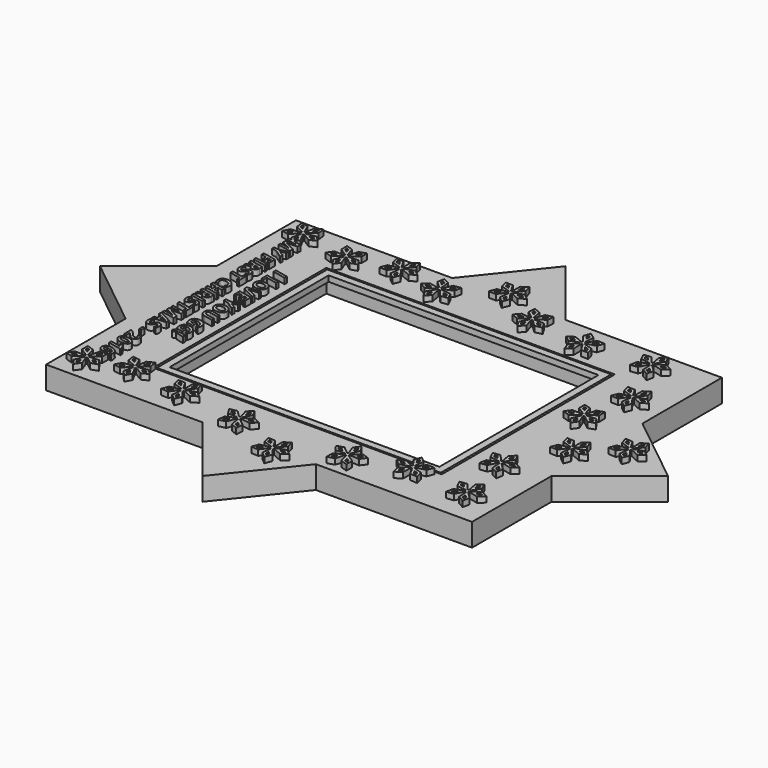
from build123d import *

# Parameters (mm, degrees)
F1_DEPTH     = 4
F4_W         = 101.6
F4_H         = 76.2
F5_DEPTH     = 8.001
F6_DEPTH     = 2
F7_TEXT_SIZE = 6.5647362641
F8_DEPTH     = 2
F9_W         = 100
F9_H         = 75
F9_W_2       = 95
F9_H_2       = 70
F10_DEPTH    = 2


# Not quite as in the source:
# - Text() gives the source's letters only with a copy of the font that has no kerning and outlines rounded to 1/6400 em; it was checked with that copy


with BuildPart() as f1:
    # F0 (on Top) → F1 (new body, symmetric)
    with BuildSketch(Plane.XY):
        Polygon((75, 20), (75, 55), (20, 55), (0, 80), (-20, 55), (-75, 55), (-75, 20), (-100, 0), (-75, -20), (-75, -55), (-20, -55), (0, -80), (20, -55), (75, -55), (75, -20), (100, 0), align=None)
    extrude(amount=F1_DEPTH, both=True)

    # F4 (on face) → F5 (cut, through all)
    with BuildSketch(Plane.XY.offset(4)):
        Rectangle(F4_W, F4_H)
    extrude(amount=-F5_DEPTH, mode=Mode.SUBTRACT)

    # F2 (on face) → F6 (join)
    with BuildSketch(Plane.XY.offset(4)):
        with BuildLine():
            Line((63.1994701679, 31.4178951368), (60.6442793174, 31.5524958216))
            Line((60.6442793174, 31.5524958216), (61.3153708432, 29.0833352779))
            Line((61.3153708432, 29.0833352779), (64.6001066479, 28.016059918))
            ThreePointArc((64.6001066479, 28.016059918), (64.5643629359, 27.8223093015), (64.5803085929, 27.6259355498))
            Line((64.5803085929, 27.6259355498), (61.2044020685, 26.8966748697))
            Line((61.2044020685, 26.8966748697), (60.2867918134, 24.5081378601))
            Line((60.2867918134, 24.5081378601), (62.8424817245, 24.3833712589))
            Line((62.8424817245, 24.3833712589), (64.8725600959, 27.1775344264))
            ThreePointArc((64.8725600959, 27.1775344264), (65.0457824678, 27.083667903), (65.237472483, 27.0381502975))
            Line((65.237472483, 27.0381502975), (64.8878281174, 23.6021184556))
            Line((64.8878281174, 23.6021184556), (66.8759046418, 21.9913207154))
            Line((66.8759046418, 21.9913207154), (67.7843163458, 24.3833712589))
            Line((67.7843163458, 24.3833712589), (65.7542379744, 27.1775344264))
            ThreePointArc((65.7542379744, 27.1775344264), (65.8970389999, 27.313272341), (65.9995642876, 27.4815146655))
            Line((65.9995642876, 27.4815146655), (69.15937871, 26.0871908808))
            Line((69.15937871, 26.0871908808), (71.3056878294, 27.480200138))
            Line((71.3056878294, 27.480200138), (69.3114272272, 29.0833352779))
            Line((69.3114272272, 29.0833352779), (66.0266914224, 28.016059918))
            ThreePointArc((66.0266914224, 28.016059918), (65.9417249379, 28.1938170862), (65.8133990352, 28.3433141666))
            Line((65.8133990352, 28.3433141666), (68.115916112, 30.9176065182))
            Line((68.115916112, 30.9176065182), (67.4543315738, 33.389331326))
            Line((67.4543315738, 33.389331326), (65.3133990352, 31.9880727875))
            Line((65.3133990352, 31.9880727875), (65.3133990352, 28.5342971722))
            ThreePointArc((65.3133990352, 28.5342971722), (65.1180858343, 28.5084192293), (64.9362507771, 28.4325711818))
            Line((64.9362507771, 28.4325711818), (63.1994701679, 31.4178951368))
        make_face()
        Polygon((62.2964551725, 25.2211391292), (61.4445585355, 25.2627279962), (61.7504286205, 26.0589069994), (63.1200942761, 26.3547811003), align=None, mode=Mode.SUBTRACT)
        Polygon((66.8188202697, 24.1229536578), (66.5160163683, 23.3256034766), (65.8533241935, 23.8625360567), (65.9951811661, 25.2565956289), align=None, mode=Mode.SUBTRACT)
        Polygon((69.2607769989, 28.0852630793), (69.9263859742, 27.5501970319), (69.2100289384, 27.0852630793), (67.9263859742, 27.6516931529), align=None, mode=Mode.SUBTRACT)
        Polygon((61.9434039514, 29.8615218975), (61.7197067761, 30.6845754121), (62.5714370596, 30.6397085171), (63.2760800154, 29.4285091956), align=None, mode=Mode.SUBTRACT)
        Polygon((66.2475713941, 31.6312506978), (66.9612155737, 32.0983368772), (67.1817437531, 31.274428608), (66.2475713941, 30.2299921593), align=None, mode=Mode.SUBTRACT)
        with BuildLine():
            Line((60.4743340463, 15.1066376163), (58.0410464334, 15.89798395))
            Line((58.0410464334, 15.89798395), (58.0502052958, 13.3392667437))
            Line((58.0502052958, 13.3392667437), (60.9467852527, 11.4582057254))
            ThreePointArc((60.9467852527, 11.4582057254), (60.8621131286, 11.2803081545), (60.8266901836, 11.0864986364))
            Line((60.8266901836, 11.0864986364), (57.3770683317, 11.2558358144))
            Line((57.3770683317, 11.2558358144), (55.8725260198, 9.1861812398))
            Line((55.8725260198, 9.1861812398), (58.3088409363, 8.404204735))
            Line((58.3088409363, 8.404204735), (60.9929287076, 10.5777361558))
            ThreePointArc((60.9929287076, 10.5777361558), (61.1359542263, 10.4422348077), (61.3093317395, 10.3486551503))
            Line((61.3093317395, 10.3486551503), (60.0822907364, 7.1201978751))
            Line((60.0822907364, 7.1201978751), (61.585720063, 5.0497346693))
            Line((61.585720063, 5.0497346693), (63.0822866263, 7.1251638173))
            Line((63.0822866263, 7.1251638173), (61.8445641408, 10.3495411293))
            ThreePointArc((61.8445641408, 10.3495411293), (62.0176308968, 10.4436942615), (62.1602070378, 10.5796683707))
            Line((62.1602070378, 10.5796683707), (64.8514758442, 8.4150348653))
            Line((64.8514758442, 8.4150348653), (67.2851885796, 9.2050728063))
            Line((67.2851885796, 9.2050728063), (65.7738026656, 11.2697350658))
            Line((65.7738026656, 11.2697350658), (62.3247603297, 11.0889784163))
            ThreePointArc((62.3247603297, 11.0889784163), (62.2886959485, 11.2826696003), (62.2034353365, 11.4602858788))
            Line((62.2034353365, 11.4602858788), (65.0937719348, 13.3509260745))
            Line((65.0937719348, 13.3509260745), (65.0944597975, 15.9096595802))
            Line((65.0944597975, 15.9096595802), (62.6638053693, 15.1102618839))
            Line((62.6638053693, 15.1102618839), (61.7699024625, 11.7741708188))
            ThreePointArc((61.7699024625, 11.7741708188), (61.5745466931, 11.7997254216), (61.379276596, 11.7735242095))
            Line((61.379276596, 11.7735242095), (60.4743340463, 15.1066376163))
        make_face()
        Polygon((57.9982500681, 9.3547484281), (57.1861450959, 9.6154072631), (57.6876591999, 10.3052921213), (59.0872324822, 10.2365889995), align=None, mode=Mode.SUBTRACT)
        Polygon((58.8582482127, 13.9283903679), (58.8551952585, 14.7812961033), (59.6662911295, 14.5175139921), (60.0334425069, 13.1652102697), align=None, mode=Mode.SUBTRACT)
        Polygon((62.0822879963, 7.1235085032), (61.5834324752, 6.4316987872), (61.0822893664, 7.1218531892), (61.5801218471, 8.4316960472), align=None, mode=Mode.SUBTRACT)
        Polygon((65.4665582086, 10.3187805964), (65.9710018247, 9.6296742031), (65.1587203012, 9.3659893347), (64.0654193012, 10.2453500178), align=None, mode=Mode.SUBTRACT)
        Polygon((63.4737942244, 14.5238166141), (64.2840123672, 14.7902825129), (64.2837830796, 13.9373713443), (63.1111218276, 13.1703048025), align=None, mode=Mode.SUBTRACT)
        with BuildLine():
            Line((54.531646123, 49.5059511711), (51.9919011994, 49.1948027344))
            Line((51.9919011994, 49.1948027344), (53.0815625657, 46.879688108))
            Line((53.0815625657, 46.879688108), (56.5017262742, 46.3990154456))
            ThreePointArc((56.5017262742, 46.3990154456), (56.5001700309, 46.2020015058), (56.5499733817, 46.0113800469))
            Line((56.5499733817, 46.0113800469), (53.3519892511, 44.7069784593))
            Line((53.3519892511, 44.7069784593), (52.8630846567, 42.1953873453))
            Line((52.8630846567, 42.1953873453), (55.4016133884, 42.5163071248))
            Line((55.4016133884, 42.5163071248), (56.9156489656, 45.6205400851))
            ThreePointArc((56.9156489656, 45.6205400851), (57.1025394512, 45.5581793543), (57.2992213136, 45.5466398853))
            Line((57.2992213136, 45.5466398853), (57.5515494993, 42.1020939809))
            Line((57.5515494993, 42.1020939809), (59.7891347663, 40.8609937433))
            Line((59.7891347663, 40.8609937433), (60.2683704375, 43.3744477011))
            Line((60.2683704375, 43.3744477011), (57.783932176, 45.773641842))
            ThreePointArc((57.783932176, 45.773641842), (57.9009930915, 45.9321147305), (57.9727458167, 46.1156044054))
            Line((57.9727458167, 46.1156044054), (61.3266773423, 45.2911595482))
            Line((61.3266773423, 45.2911595482), (63.1984856844, 47.035708532))
            Line((63.1984856844, 47.035708532), (60.9561408862, 48.2681887276))
            Line((60.9561408862, 48.2681887276), (57.9066380204, 46.6467392919))
            ThreePointArc((57.9066380204, 46.6467392919), (57.7920951594, 46.8070416542), (57.6397589199, 46.9319839788))
            Line((57.6397589199, 46.9319839788), (59.460274413, 49.8669949397))
            Line((59.460274413, 49.8669949397), (58.3795303219, 52.1862857442))
            Line((58.3795303219, 52.1862857442), (56.5144493508, 50.4345464378))
            Line((56.5144493508, 50.4345464378), (57.1141911925, 47.0332414346))
            ThreePointArc((57.1141911925, 47.0332414346), (56.9263388957, 46.9738408544), (56.7604371968, 46.8675697828))
            Line((56.7604371968, 46.8675697828), (54.531646123, 49.5059511711))
        make_face()
        Polygon((59.3627634581, 42.9503297944), (59.2030182344, 42.1125118084), (58.4571564787, 42.5262118876), (58.3547824209, 43.9237257673), align=None, mode=Mode.SUBTRACT)
        Polygon((54.7184053426, 43.246530903), (53.8722290987, 43.1395576431), (54.0351972969, 43.9767546812), (55.3326766551, 44.5059737347), align=None, mode=Mode.SUBTRACT)
        Polygon((53.5649237515, 47.755109129), (53.201703296, 48.5268140045), (54.0482849372, 48.6305301501), (54.9525453381, 47.560091633), align=None, mode=Mode.SUBTRACT)
        Polygon((57.4963910382, 50.2453626051), (58.1180846952, 50.8292757072), (58.4783327256, 50.0561787724), (57.7397170299, 48.8653923324), align=None, mode=Mode.SUBTRACT)
        Polygon((61.0795735671, 47.2764841685), (61.8279836906, 46.8651287623), (61.2032446614, 46.2828641073), (59.8407435681, 46.6177865738), align=None, mode=Mode.SUBTRACT)
        with BuildLine():
            Line((69.176194365, -2.7749478988), (66.6210035146, -2.640347214))
            Line((66.6210035146, -2.640347214), (67.2920950403, -5.1095077577))
            Line((67.2920950403, -5.1095077577), (70.5768308451, -6.1767831176))
            ThreePointArc((70.5768308451, -6.1767831176), (70.5410871331, -6.3705337341), (70.5570327901, -6.5669074858))
            Line((70.5570327901, -6.5669074858), (67.1811262657, -7.2961681658))
            Line((67.1811262657, -7.2961681658), (66.2635160106, -9.6847051755))
            Line((66.2635160106, -9.6847051755), (68.8192059217, -9.8094717767))
            Line((68.8192059217, -9.8094717767), (70.8492842931, -7.0153086091))
            ThreePointArc((70.8492842931, -7.0153086091), (71.022506665, -7.1091751326), (71.2141966802, -7.1546927381))
            Line((71.2141966802, -7.1546927381), (70.8645523146, -10.59072458))
            Line((70.8645523146, -10.59072458), (72.852628839, -12.2015223202))
            Line((72.852628839, -12.2015223202), (73.761040543, -9.8094717767))
            Line((73.761040543, -9.8094717767), (71.7309621716, -7.0153086091))
            ThreePointArc((71.7309621716, -7.0153086091), (71.8737631971, -6.8795706945), (71.9762884848, -6.7113283701))
            Line((71.9762884848, -6.7113283701), (75.1361029072, -8.1056521548))
            Line((75.1361029072, -8.1056521548), (77.2824120266, -6.7126428976))
            Line((77.2824120266, -6.7126428976), (75.2881514244, -5.1095077577))
            Line((75.2881514244, -5.1095077577), (72.0034156196, -6.1767831176))
            ThreePointArc((72.0034156196, -6.1767831176), (71.9184491351, -5.9990259494), (71.7901232323, -5.849528869))
            Line((71.7901232323, -5.849528869), (74.0926403092, -3.2752365174))
            Line((74.0926403092, -3.2752365174), (73.431055771, -0.8035117096))
            Line((73.431055771, -0.8035117096), (71.2901232323, -2.204770248))
            Line((71.2901232323, -2.204770248), (71.2901232323, -5.6585458634))
            ThreePointArc((71.2901232323, -5.6585458634), (71.0948100315, -5.6844238063), (70.9129749743, -5.7602718538))
            Line((70.9129749743, -5.7602718538), (69.176194365, -2.7749478988))
        make_face()
        Polygon((68.2731793697, -8.9717039064), (67.4212827327, -8.9301150393), (67.7271528177, -8.1339360361), (69.0968184732, -7.8380619353), align=None, mode=Mode.SUBTRACT)
        Polygon((67.9201281486, -4.3313211381), (67.6964309733, -3.5082676235), (68.5481612568, -3.5531345184), (69.2528042126, -4.76433384), align=None, mode=Mode.SUBTRACT)
        Polygon((72.7955444668, -10.0698893778), (72.4927405655, -10.867239559), (71.8300483907, -10.3303069789), (71.9719053633, -8.9362474067), align=None, mode=Mode.SUBTRACT)
        Polygon((75.237501196, -6.1075799563), (75.9031101714, -6.6426460036), (75.1867531355, -7.1075799563), (73.9031101714, -6.5411498826), align=None, mode=Mode.SUBTRACT)
        Polygon((72.2242955913, -2.5615923378), (72.9379397709, -2.0945061583), (73.1584679503, -2.9184144276), (72.2242955913, -3.9628508763), align=None, mode=Mode.SUBTRACT)
        with BuildLine():
            Line((58.7020704823, -22.0312884666), (56.1623255587, -22.3424369034))
            Line((56.1623255587, -22.3424369034), (57.2519869251, -24.6575515297))
            Line((57.2519869251, -24.6575515297), (60.6721506335, -25.1382241921))
            ThreePointArc((60.6721506335, -25.1382241921), (60.6705943902, -25.3352381319), (60.720397741, -25.5258595908))
            Line((60.720397741, -25.5258595908), (57.5224136105, -26.8302611784))
            Line((57.5224136105, -26.8302611784), (57.033509016, -29.3418522924))
            Line((57.033509016, -29.3418522924), (59.5720377477, -29.0209325129))
            Line((59.5720377477, -29.0209325129), (61.086073325, -25.9166995526))
            ThreePointArc((61.086073325, -25.9166995526), (61.2729638106, -25.9790602834), (61.469645673, -25.9905997524))
            Line((61.469645673, -25.9905997524), (61.7219738586, -29.4351456568))
            Line((61.7219738586, -29.4351456568), (63.9595591256, -30.6762458944))
            Line((63.9595591256, -30.6762458944), (64.4387947969, -28.1627919366))
            Line((64.4387947969, -28.1627919366), (61.9543565353, -25.7635977957))
            ThreePointArc((61.9543565353, -25.7635977957), (62.0714174509, -25.6051249072), (62.143170176, -25.4216352323))
            Line((62.143170176, -25.4216352323), (65.4971017016, -26.2460800895))
            Line((65.4971017016, -26.2460800895), (67.3689100438, -24.5015311057))
            Line((67.3689100438, -24.5015311057), (65.1265652456, -23.2690509101))
            Line((65.1265652456, -23.2690509101), (62.0770623797, -24.8905003458))
            ThreePointArc((62.0770623797, -24.8905003458), (61.9625195187, -24.7301979835), (61.8101832792, -24.6052556589))
            Line((61.8101832792, -24.6052556589), (63.6306987723, -21.670244698))
            Line((63.6306987723, -21.670244698), (62.5499546812, -19.3509538935))
            Line((62.5499546812, -19.3509538935), (60.6848737102, -21.1026932))
            Line((60.6848737102, -21.1026932), (61.2846155518, -24.5039982031))
            ThreePointArc((61.2846155518, -24.5039982031), (61.096763255, -24.5633987833), (60.9308615561, -24.6696698549))
            Line((60.9308615561, -24.6696698549), (58.7020704823, -22.0312884666))
        make_face()
        Polygon((58.888829702, -28.2907087347), (58.0426534581, -28.3976819946), (58.2056216562, -27.5604849566), (59.5031010144, -27.031265903), align=None, mode=Mode.SUBTRACT)
        Polygon((63.5331878175, -28.5869098433), (63.3734425937, -29.4247278293), (62.627580838, -29.0110277501), (62.5252067802, -27.6135138704), align=None, mode=Mode.SUBTRACT)
        Polygon((65.2499979265, -24.2607554692), (65.99840805, -24.6721108754), (65.3736690207, -25.2543755304), (64.0111679275, -24.9194530639), align=None, mode=Mode.SUBTRACT)
        Polygon((57.7353481108, -23.7821305087), (57.3721276554, -23.0104256332), (58.2187092966, -22.9067094876), (59.1229696975, -23.9771480047), align=None, mode=Mode.SUBTRACT)
        Polygon((61.6668153975, -21.2918770327), (62.2885090546, -20.7079639305), (62.6487570849, -21.4810608653), (61.9101413892, -22.6718473053), align=None, mode=Mode.SUBTRACT)
        with BuildLine():
            Line((62.2558930258, -41.1344152125), (59.7161481023, -41.4455636493))
            Line((59.7161481023, -41.4455636493), (60.8058094686, -43.7606782757))
            Line((60.8058094686, -43.7606782757), (64.225973177, -44.2413509381))
            ThreePointArc((64.225973177, -44.2413509381), (64.2244169338, -44.4383648779), (64.2742202845, -44.6289863368))
            Line((64.2742202845, -44.6289863368), (61.076236154, -45.9333879244))
            Line((61.076236154, -45.9333879244), (60.5873315596, -48.4449790384))
            Line((60.5873315596, -48.4449790384), (63.1258602913, -48.1240592589))
            Line((63.1258602913, -48.1240592589), (64.6398958685, -45.0198262986))
            ThreePointArc((64.6398958685, -45.0198262986), (64.8267863541, -45.0821870294), (65.0234682165, -45.0937264984))
            Line((65.0234682165, -45.0937264984), (65.2757964021, -48.5382724028))
            Line((65.2757964021, -48.5382724028), (67.5133816691, -49.7793726404))
            Line((67.5133816691, -49.7793726404), (67.9926173404, -47.2659186826))
            Line((67.9926173404, -47.2659186826), (65.5081790789, -44.8667245417))
            ThreePointArc((65.5081790789, -44.8667245417), (65.6252399944, -44.7082516532), (65.6969927195, -44.5247619783))
            Line((65.6969927195, -44.5247619783), (69.0509242452, -45.3492068355))
            Line((69.0509242452, -45.3492068355), (70.9227325873, -43.6046578517))
            Line((70.9227325873, -43.6046578517), (68.6803877891, -42.3721776561))
            Line((68.6803877891, -42.3721776561), (65.6308849232, -43.9936270918))
            ThreePointArc((65.6308849232, -43.9936270918), (65.5163420622, -43.8333247295), (65.3640058227, -43.7083824049))
            Line((65.3640058227, -43.7083824049), (67.1845213159, -40.773371444))
            Line((67.1845213159, -40.773371444), (66.1037772248, -38.4540806395))
            Line((66.1037772248, -38.4540806395), (64.2386962537, -40.2058199459))
            Line((64.2386962537, -40.2058199459), (64.8384380953, -43.6071249491))
            ThreePointArc((64.8384380953, -43.6071249491), (64.6505857985, -43.6665255293), (64.4846840997, -43.7727966009))
            Line((64.4846840997, -43.7727966009), (62.2558930258, -41.1344152125))
        make_face()
        Polygon((62.4426522455, -47.3938354807), (61.5964760016, -47.5008087405), (61.7594441997, -46.6636117025), (63.0569235579, -46.134392649), align=None, mode=Mode.SUBTRACT)
        Polygon((67.087010361, -47.6900365893), (66.9272651372, -48.5278545752), (66.1814033816, -48.1141544961), (66.0790293237, -46.7166406164), align=None, mode=Mode.SUBTRACT)
        Polygon((61.2891706543, -42.8852572547), (60.9259501989, -42.1135523792), (61.7725318401, -42.0098362336), (62.676792241, -43.0802747507), align=None, mode=Mode.SUBTRACT)
        Polygon((68.80382047, -43.3638822152), (69.5522305935, -43.7752376214), (68.9274915642, -44.3575022764), (67.564990471, -44.0225798099), align=None, mode=Mode.SUBTRACT)
        Polygon((65.2206379411, -40.3950037786), (65.8423315981, -39.8110906765), (66.2025796285, -40.5841876113), (65.4639639327, -41.7749740513), align=None, mode=Mode.SUBTRACT)
        with BuildLine():
            Line((30.7487925384, 45.8431862279), (28.6434021146, 44.389071793))
            Line((28.6434021146, 44.389071793), (30.6829098604, 42.8439097363))
            Line((30.6829098604, 42.8439097363), (33.9356177001, 44.0051408548))
            ThreePointArc((33.9356177001, 44.0051408548), (34.0256574679, 43.8298988662), (34.1582266087, 43.6841513542))
            Line((34.1582266087, 43.6841513542), (31.9306403958, 41.0447526224))
            Line((31.9306403958, 41.0447526224), (32.6629839838, 38.5930612683))
            Line((32.6629839838, 38.5930612683), (34.7627629801, 40.0552670655))
            Line((34.7627629801, 40.0552670655), (34.6635085582, 43.507616202))
            ThreePointArc((34.6635085582, 43.507616202), (34.8579974118, 43.5390963573), (35.0375776502, 43.6201386444))
            Line((35.0375776502, 43.6201386444), (36.8594330169, 40.685959198))
            Line((36.8594330169, 40.685959198), (39.4174366696, 40.6248450461))
            Line((39.4174366696, 40.6248450461), (38.6756637124, 43.0736999839))
            Line((38.6756637124, 43.0736999839), (35.3616132664, 44.0461379729))
            ThreePointArc((35.3616132664, 44.0461379729), (35.3917742205, 44.2408357675), (35.3701917709, 44.4366701674))
            Line((35.3701917709, 44.4366701674), (38.723746523, 45.2626462722))
            Line((38.723746523, 45.2626462722), (39.5723361357, 47.6765670032))
            Line((39.5723361357, 47.6765670032), (37.0141162398, 47.7278367912))
            Line((37.0141162398, 47.7278367912), (35.0651748457, 44.8764873838))
            ThreePointArc((35.0651748457, 44.8764873838), (34.8893264869, 44.965337083), (34.696407561, 45.0053271113))
            Line((34.696407561, 45.0053271113), (34.9471630142, 48.4499878644))
            Line((34.9471630142, 48.4499878644), (32.9136165847, 50.0029870742))
            Line((32.9136165847, 50.0029870742), (32.0743226956, 47.5858186079))
            Line((32.0743226956, 47.5858186079), (34.1838611179, 44.8511497713))
            ThreePointArc((34.1838611179, 44.8511497713), (34.0450199012, 44.7113641108), (33.9473718975, 44.5402449075))
            Line((33.9473718975, 44.5402449075), (30.7487925384, 45.8431862279))
        make_face()
        Polygon((33.8187221186, 40.3850955844), (33.1187957865, 39.8976936521), (32.8746812572, 40.7149241034), (33.7784528245, 41.7857753749), align=None, mode=Mode.SUBTRACT)
        Polygon((30.7048707531, 43.8436685669), (30.0250348378, 44.3587225857), (30.7268316457, 44.8434273974), (32.0245524988, 44.3148008004), align=None, mode=Mode.SUBTRACT)
        Polygon((38.0702534806, 42.2777863886), (38.317511133, 41.4615014093), (37.4648432488, 41.4818727933), (36.7256839423, 42.6723218729), align=None, mode=Mode.SUBTRACT)
        Polygon((33.0319361351, 47.8738750267), (33.3117007648, 48.6795978488), (33.9895495747, 48.1619314455), (33.8878136025, 46.7643709697), align=None, mode=Mode.SUBTRACT)
        Polygon((37.5836263266, 46.9066353419), (38.4374636444, 46.8895234203), (38.1542364363, 46.0838477215), (36.7918884035, 45.7483032009), align=None, mode=Mode.SUBTRACT)
        with BuildLine():
            Line((-1.8873223392, 59.0391116046), (-4.4425131897, 59.1737122894))
            Line((-4.4425131897, 59.1737122894), (-3.7714216639, 56.7045517457))
            Line((-3.7714216639, 56.7045517457), (-0.4866858591, 55.6372763858))
            ThreePointArc((-0.4866858591, 55.6372763858), (-0.5224295712, 55.4435257693), (-0.5064839142, 55.2471520176))
            Line((-0.5064839142, 55.2471520176), (-3.8823904386, 54.5178913375))
            Line((-3.8823904386, 54.5178913375), (-4.8000006936, 52.1293543279))
            Line((-4.8000006936, 52.1293543279), (-2.2443107825, 52.0045877267))
            Line((-2.2443107825, 52.0045877267), (-0.2142324111, 54.7987508942))
            ThreePointArc((-0.2142324111, 54.7987508942), (-0.0410100392, 54.7048843708), (0.150679976, 54.6593667653))
            Line((0.150679976, 54.6593667653), (-0.1989643897, 51.2233349234))
            Line((-0.1989643897, 51.2233349234), (1.7891121347, 49.6125371832))
            Line((1.7891121347, 49.6125371832), (2.6975238387, 52.0045877267))
            Line((2.6975238387, 52.0045877267), (0.6674454673, 54.7987508942))
            ThreePointArc((0.6674454673, 54.7987508942), (0.8102464928, 54.9344888088), (0.9127717805, 55.1027311333))
            Line((0.9127717805, 55.1027311333), (4.072586203, 53.7084073486))
            Line((4.072586203, 53.7084073486), (6.2188953224, 55.1014166058))
            Line((6.2188953224, 55.1014166058), (4.2246347201, 56.7045517457))
            Line((4.2246347201, 56.7045517457), (0.9398989153, 55.6372763858))
            ThreePointArc((0.9398989153, 55.6372763858), (0.8549324308, 55.815033554), (0.7266065281, 55.9645306344))
            Line((0.7266065281, 55.9645306344), (3.029123605, 58.538822986))
            Line((3.029123605, 58.538822986), (2.3675390667, 61.0105477938))
            Line((2.3675390667, 61.0105477938), (0.2266065281, 59.6092892553))
            Line((0.2266065281, 59.6092892553), (0.2266065281, 56.15551364))
            ThreePointArc((0.2266065281, 56.15551364), (0.0312933273, 56.1296356971), (-0.1505417299, 56.0537876496))
            Line((-0.1505417299, 56.0537876496), (-1.8873223392, 59.0391116046))
        make_face()
        Polygon((1.7320277626, 51.7441701256), (1.4292238613, 50.9468199444), (0.7665316865, 51.4837525245), (0.9083886591, 52.8778120967), align=None, mode=Mode.SUBTRACT)
        Polygon((-2.7903373345, 52.842355597), (-3.6422339716, 52.883944464), (-3.3363638866, 53.6801234673), (-1.966698231, 53.9759975681), align=None, mode=Mode.SUBTRACT)
        Polygon((-3.1433885557, 57.4827383653), (-3.3670857309, 58.3057918799), (-2.5153554474, 58.2609249849), (-1.8107124917, 57.0497256634), align=None, mode=Mode.SUBTRACT)
        Polygon((4.1739844918, 55.7064795471), (4.8395934672, 55.1714134997), (4.1232364313, 54.7064795471), (2.8395934672, 55.2729096207), align=None, mode=Mode.SUBTRACT)
        Polygon((1.1607788871, 59.2524671656), (1.8744230666, 59.719553345), (2.094951246, 58.8956450758), (1.1607788871, 57.8512086271), align=None, mode=Mode.SUBTRACT)
        with BuildLine():
            Line((10.6080443368, 47.3445019694), (8.9370155178, 45.406776418))
            Line((8.9370155178, 45.406776418), (11.3000724022, 44.4254101317))
            Line((11.3000724022, 44.4254101317), (14.1551981912, 46.3688150637))
            ThreePointArc((14.1551981912, 46.3688150637), (14.2864914397, 46.2219171493), (14.4515093583, 46.1142788621))
            Line((14.4515093583, 46.1142788621), (12.9609066139, 42.9987260284))
            Line((12.9609066139, 42.9987260284), (14.2874168232, 40.8106930554))
            Line((14.2874168232, 40.8106930554), (15.9509763606, 42.7548348435))
            Line((15.9509763606, 42.7548348435), (14.9849708261, 46.070765981))
            ThreePointArc((14.9849708261, 46.070765981), (15.1652508899, 46.1502393284), (15.3186143255, 46.2739186353))
            Line((15.3186143255, 46.2739186353), (17.82105957, 43.8935124095))
            Line((17.82105957, 43.8935124095), (20.3119167847, 44.4789592151))
            Line((20.3119167847, 44.4789592151), (18.9769962368, 46.6618712053))
            Line((18.9769962368, 46.6618712053), (15.5248461941, 46.7678244207))
            ThreePointArc((15.5248461941, 46.7678244207), (15.5049721525, 46.9638395651), (15.4347380497, 47.1479158676))
            Line((15.4347380497, 47.1479158676), (18.4719370102, 48.7922967467))
            Line((18.4719370102, 48.7922967467), (18.6848612208, 51.3421557442))
            Line((18.6848612208, 51.3421557442), (16.1962754125, 50.7471277605))
            Line((16.1962754125, 50.7471277605), (15.0287348863, 47.4966793113))
            ThreePointArc((15.0287348863, 47.4966793113), (14.8361719894, 47.5383499854), (14.639401491, 47.52843609))
            Line((14.639401491, 47.52843609), (14.0140484347, 50.9251255895))
            Line((14.0140484347, 50.9251255895), (11.6547856191, 51.9155783109))
            Line((11.6547856191, 51.9155783109), (11.4516755536, 49.3649188025))
            Line((11.4516755536, 49.3649188025), (14.1822458679, 47.2500779669))
            ThreePointArc((14.1822458679, 47.2500779669), (14.0831094942, 47.0798167154), (14.031732741, 46.8896132886))
            Line((14.031732741, 46.8896132886), (10.6080443368, 47.3445019694))
        make_face()
        Polygon((14.954286445, 42.8361319051), (14.3997665992, 42.1880846424), (13.9575965295, 42.9174289668), (14.5623607225, 44.1814644736), align=None, mode=Mode.SUBTRACT)
        Polygon((18.5916840145, 45.7390849401), (19.0366575305, 45.01144761), (18.2063717922, 44.8162986748), (17.191085, 45.7820720545), align=None, mode=Mode.SUBTRACT)
        Polygon((11.0693963804, 45.3984407443), (10.2817107522, 45.7255628397), (10.8387203586, 46.3714713568), (12.2277719774, 46.1869148833), align=None, mode=Mode.SUBTRACT)
        Polygon((12.3057998473, 49.8849877315), (12.3735032025, 50.7352075676), (13.159924141, 50.4050566605), (13.4136410605, 49.0269589802), align=None, mode=Mode.SUBTRACT)
        Polygon((16.954341204, 50.0959366865), (17.7849372897, 50.294534586), (17.7138712187, 49.4434878207), (16.480039558, 48.7754745567), align=None, mode=Mode.SUBTRACT)
        with BuildLine():
            Line((22.2884685802, -45.2107591539), (19.8413384478, -45.9582026245))
            Line((19.8413384478, -45.9582026245), (21.3164608455, -48.0489277471))
            Line((21.3164608455, -48.0489277471), (24.7681325141, -47.9283927164))
            ThreePointArc((24.7681325141, -47.9283927164), (24.8008110252, -48.1226838105), (24.8829588202, -48.3017610401))
            Line((24.8829588202, -48.3017610401), (21.960066213, -50.141669953))
            Line((21.960066213, -50.141669953), (21.9147223979, -52.7000017464))
            Line((21.9147223979, -52.7000017464), (24.3589580393, -51.9431465712))
            Line((24.3589580393, -51.9431465712), (25.3109476175, -48.6231643659))
            ThreePointArc((25.3109476175, -48.6231643659), (25.5058276439, -48.6521245048), (25.7015252746, -48.6293352163))
            Line((25.7015252746, -48.6293352163), (26.5481591473, -51.977734399))
            Line((26.5481591473, -51.977734399), (28.9672652608, -52.8114269312))
            Line((28.9672652608, -52.8114269312), (29.002763566, -50.2529395858))
            Line((29.002763566, -50.2529395858), (26.1394538137, -48.3216127715))
            ThreePointArc((26.1394538137, -48.3216127715), (26.2272177826, -48.1452200276), (26.266017775, -47.9520582432))
            Line((26.266017775, -47.9520582432), (29.7121588915, -48.181573833))
            Line((29.7121588915, -48.181573833), (31.2525925071, -46.1384923607))
            Line((31.2525925071, -46.1384923607), (28.8302960249, -45.3141153966))
            Line((28.8302960249, -45.3141153966), (26.1086836995, -47.4404719874))
            ThreePointArc((26.1086836995, -47.4404719874), (25.9680447889, -47.3024951373), (25.7963268722, -47.2059038777))
            Line((25.7963268722, -47.2059038777), (27.0795253395, -43.9993531305))
            Line((27.0795253395, -43.9993531305), (25.6124595579, -41.9029668066))
            Line((25.6124595579, -41.9029668066), (24.0798996959, -43.9519611687))
            Line((24.0798996959, -43.9519611687), (25.2611605268, -47.1974486283))
            ThreePointArc((25.2611605268, -47.1974486283), (25.086476931, -47.2885669892), (24.9415494296, -47.4220320921))
            Line((24.9415494296, -47.4220320921), (22.2884685802, -45.2107591539))
        make_face()
        Polygon((23.5593274305, -51.3426543652), (22.7445822167, -51.5949394236), (22.7596968218, -50.7421621591), (23.9455666289, -49.9956782061), align=None, mode=Mode.SUBTRACT)
        Polygon((28.1845620931, -50.8278711902), (28.1727293247, -51.6807003053), (27.3663606202, -51.4028027946), (27.0228661159, -50.0442973596), align=None, mode=Mode.SUBTRACT)
        Polygon((21.6404634237, -47.1028715494), (21.1487559579, -46.4059631752), (21.964466002, -46.1568153516), (23.0408683533, -47.0539683316), align=None, mode=Mode.SUBTRACT)
        Polygon((29.1240611756, -46.269319875), (29.9325323843, -46.5444658142), (29.4183937409, -47.2263693547), (28.0184334248, -47.1331309449), align=None, mode=Mode.SUBTRACT)
        Polygon((25.0797749104, -43.9677584893), (25.5906281977, -43.2847603686), (26.0796501249, -43.9835558099), (25.5590335566, -45.2845107977), align=None, mode=Mode.SUBTRACT)
        with BuildLine():
            Line((-16.6277704817, 48.9843288177), (-18.8866751393, 50.1861887822))
            Line((-18.8866751393, 50.1861887822), (-19.3219720007, 47.6647538199))
            Line((-19.3219720007, 47.6647538199), (-16.7960404198, 45.3092845142))
            ThreePointArc((-16.7960404198, 45.3092845142), (-16.9103177732, 45.1487927672), (-16.9788572336, 44.964078781))
            Line((-16.9788572336, 44.964078781), (-20.346666486, 45.729863895))
            Line((-20.346666486, 45.729863895), (-22.1877431647, 43.9529130545))
            Line((-22.1877431647, 43.9529130545), (-19.9242301412, 42.7597548845))
            Line((-19.9242301412, 42.7597548845), (-16.903489924, 44.434178529))
            ThreePointArc((-16.903489924, 44.434178529), (-16.7861668464, 44.2758996301), (-16.6316732642, 44.1536349688))
            Line((-16.6316732642, 44.1536349688), (-18.4006884799, 41.187298648))
            Line((-18.4006884799, 41.187298648), (-17.2796317855, 38.8872226678))
            Line((-17.2796317855, 38.8872226678), (-15.4454069417, 40.671245327))
            Line((-15.4454069417, 40.671245327), (-16.1044183971, 44.0615653566))
            ThreePointArc((-16.1044183971, 44.0615653566), (-15.9176313942, 44.1242353644), (-15.7536096489, 44.2333856343))
            Line((-15.7536096489, 44.2333856343), (-13.4791119264, 41.6343038519))
            Line((-13.4791119264, 41.6343038519), (-10.9451841072, 41.9897295599))
            Line((-10.9451841072, 41.9897295599), (-12.0750838343, 44.2854743701))
            Line((-12.0750838343, 44.2854743701), (-15.5031155299, 44.7063837366))
            ThreePointArc((-15.5031155299, 44.7063837366), (-15.504997891, 44.9033948303), (-15.5581204597, 45.0931180684))
            Line((-15.5581204597, 45.0931180684), (-12.3833883442, 46.4531335081))
            Line((-12.3833883442, 46.4531335081), (-11.9383915213, 48.9728746563))
            Line((-11.9383915213, 48.9728746563), (-14.4709328003, 48.6077003193))
            Line((-14.4709328003, 48.6077003193), (-15.9305614473, 45.4775165844))
            ThreePointArc((-15.9305614473, 45.4775165844), (-16.1185118134, 45.5366061287), (-16.3153651117, 45.5447112684))
            Line((-16.3153651117, 45.5447112684), (-16.6277704817, 48.9843288177))
        make_face()
        Polygon((-16.4305007877, 40.8432631007), (-17.041909069, 40.2485888809), (-17.4155946338, 41.0152808743), (-16.6978735217, 42.218776573), align=None, mode=Mode.SUBTRACT)
        Polygon((-20.0650422561, 43.7497912213), (-20.8195465973, 44.1475106113), (-20.2058543711, 44.7398275582), (-18.8394739236, 44.4291348412), align=None, mode=Mode.SUBTRACT)
        Polygon((-12.5427920682, 43.4023194759), (-12.1656741536, 42.6360864425), (-13.0114036924, 42.517458746), (-13.9353956134, 43.5733096907), align=None, mode=Mode.SUBTRACT)
        Polygon((-18.4239048277, 48.1046121525), (-18.2788058739, 48.9450904732), (-17.5258376547, 48.5444704851), (-17.3990892086, 47.1489561272), align=None, mode=Mode.SUBTRACT)
        Polygon((-13.7750846483, 47.8895113822), (-12.9309042219, 48.0112361612), (-13.0792364963, 47.1713224452), (-14.3672820961, 46.6195398572), align=None, mode=Mode.SUBTRACT)
        with BuildLine():
            Line((-14.2098443098, -46.6718334562), (-16.7128063641, -47.2031512344))
            Line((-16.7128063641, -47.2031512344), (-15.4255159534, -49.414485905))
            Line((-15.4255159534, -49.414485905), (-11.9764736175, -49.5952425545))
            ThreePointArc((-11.9764736175, -49.5952425545), (-11.9608530426, -49.7916424322), (-11.8946254538, -49.9771978709))
            Line((-11.8946254538, -49.9771978709), (-14.9667542, -51.5553584988))
            Line((-14.9667542, -51.5553584988), (-15.2348987758, -54.1000030935))
            Line((-15.2348987758, -54.1000030935), (-12.7339999141, -53.5590571535))
            Line((-12.7339999141, -53.5590571535), (-11.4962774286, -50.3346798415))
            ThreePointArc((-11.4962774286, -50.3346798415), (-11.304663022, -50.3805146919), (-11.1077238624, -50.3748682959))
            Line((-11.1077238624, -50.3748682959), (-10.556143905, -53.7843148128))
            Line((-10.556143905, -53.7843148128), (-8.2189043125, -54.8256738833))
            Line((-8.2189043125, -54.8256738833), (-7.9605542241, -52.2800162358))
            Line((-7.9605542241, -52.2800162358), (-10.6446419954, -50.1064848149))
            ThreePointArc((-10.6446419954, -50.1064848149), (-10.5418383543, -49.9384124326), (-10.4863508488, -49.7493673293))
            Line((-10.4863508488, -49.7493673293), (-7.0733269413, -50.2783605316))
            Line((-7.0733269413, -50.2783605316), (-5.3606888575, -48.377311237))
            Line((-5.3606888575, -48.377311237), (-7.7019185836, -47.3449542271))
            Line((-7.7019185836, -47.3449542271), (-10.5984985405, -49.2260152454))
            ThreePointArc((-10.5984985405, -49.2260152454), (-10.7265768028, -49.0763059502), (-10.889222798, -48.9651160469))
            Line((-10.889222798, -48.9651160469), (-9.3314379762, -45.8826053089))
            Line((-9.3314379762, -45.8826053089), (-10.6102090225, -43.66633316))
            Line((-10.6102090225, -43.66633316), (-12.3155186571, -45.5739590869))
            Line((-12.3155186571, -45.5739590869), (-11.4216157503, -48.9100501519))
            ThreePointArc((-11.4216157503, -48.9100501519), (-11.6035761107, -48.9855971014), (-11.7595843694, -49.1059230653))
            Line((-11.7595843694, -49.1059230653), (-14.2098443098, -46.6718334562))
        make_face()
        Polygon((-13.4782513427, -52.891157602), (-14.3118842966, -53.0714729153), (-14.2225027714, -52.2232580504), (-12.9760851935, -51.582970058), align=None, mode=Mode.SUBTRACT)
        Polygon((-15.0202920722, -48.5002684221), (-15.4493888758, -47.7631568652), (-14.615068191, -47.5860509391), (-13.6209539099, -48.5736046276), align=None, mode=Mode.SUBTRACT)
        Polygon((-8.8257507844, -52.7814490948), (-8.9118674805, -53.630001644), (-9.6909473447, -53.2828819538), (-9.9147331985, -51.8996085234), align=None, mode=Mode.SUBTRACT)
        Polygon((-7.4925228539, -48.3221271839), (-6.7111086709, -48.6666890184), (-7.2827226711, -49.3011875748), (-8.6692294526, -49.0862893841), align=None, mode=Mode.SUBTRACT)
        Polygon((-11.3208250968, -45.6768411609), (-10.7523885519, -45.0409658519), (-10.3261315365, -45.7797232349), (-10.9581526999, -47.0303529725), align=None, mode=Mode.SUBTRACT)
        with BuildLine():
            Line((-49.6192632764, 48.0343491106), (-52.0525508893, 48.8256954442))
            Line((-52.0525508893, 48.8256954442), (-52.0433920269, 46.266978238))
            Line((-52.0433920269, 46.266978238), (-49.14681207, 44.3859172197))
            ThreePointArc((-49.14681207, 44.3859172197), (-49.2314841941, 44.2080196487), (-49.2669071391, 44.0142101306))
            Line((-49.2669071391, 44.0142101306), (-52.716528991, 44.1835473087))
            Line((-52.716528991, 44.1835473087), (-54.2210713029, 42.1138927341))
            Line((-54.2210713029, 42.1138927341), (-51.7847563864, 41.3319162293))
            Line((-51.7847563864, 41.3319162293), (-49.1006686151, 43.5054476501))
            ThreePointArc((-49.1006686151, 43.5054476501), (-48.9576430964, 43.369946302), (-48.7842655832, 43.2763666446))
            Line((-48.7842655832, 43.2763666446), (-50.0113065863, 40.0479093694))
            Line((-50.0113065863, 40.0479093694), (-48.5078772597, 37.9774461636))
            Line((-48.5078772597, 37.9774461636), (-47.0113106964, 40.0528753115))
            Line((-47.0113106964, 40.0528753115), (-48.2490331819, 43.2772526235))
            ThreePointArc((-48.2490331819, 43.2772526235), (-48.0759664259, 43.3714057558), (-47.9333902849, 43.507379865))
            Line((-47.9333902849, 43.507379865), (-45.2421214785, 41.3427463596))
            Line((-45.2421214785, 41.3427463596), (-42.8084087431, 42.1327843006))
            Line((-42.8084087431, 42.1327843006), (-44.3197946571, 44.1974465601))
            Line((-44.3197946571, 44.1974465601), (-47.768836993, 44.0166899106))
            ThreePointArc((-47.768836993, 44.0166899106), (-47.8049013742, 44.2103810946), (-47.8901619862, 44.387997373))
            Line((-47.8901619862, 44.387997373), (-44.9998253879, 46.2786375687))
            Line((-44.9998253879, 46.2786375687), (-44.9991375252, 48.8373710745))
            Line((-44.9991375252, 48.8373710745), (-47.4297919534, 48.0379733782))
            Line((-47.4297919534, 48.0379733782), (-48.3236948602, 44.7018823131))
            ThreePointArc((-48.3236948602, 44.7018823131), (-48.5190506296, 44.7274369159), (-48.7143207267, 44.7012357037))
            Line((-48.7143207267, 44.7012357037), (-49.6192632764, 48.0343491106))
        make_face()
        Polygon((-48.0113093264, 40.0512199975), (-48.5101648475, 39.3594102815), (-49.0113079563, 40.0495646834), (-48.5134754756, 41.3594075414), align=None, mode=Mode.SUBTRACT)
        Polygon((-52.0953472546, 42.2824599224), (-52.9074522268, 42.5431187573), (-52.4059381228, 43.2330036156), (-51.0063648405, 43.1643004938), align=None, mode=Mode.SUBTRACT)
        Polygon((-44.6270391141, 43.2464920907), (-44.122595498, 42.5573856973), (-44.9348770215, 42.293700829), (-46.0281780215, 43.1730615121), align=None, mode=Mode.SUBTRACT)
        Polygon((-51.23534911, 46.8561018622), (-51.2384020642, 47.7090075976), (-50.4273061932, 47.4452254864), (-50.0601548158, 46.092921764), align=None, mode=Mode.SUBTRACT)
        Polygon((-46.6198030983, 47.4515281084), (-45.8095849555, 47.7179940071), (-45.8098142431, 46.8650828386), (-46.9824754951, 46.0980162968), align=None, mode=Mode.SUBTRACT)
        with BuildLine():
            Line((-63.0006898596, 49.990476524), (-63.3118382963, 52.5302214476))
            Line((-63.3118382963, 52.5302214476), (-65.6269529227, 51.4405600812))
            Line((-65.6269529227, 51.4405600812), (-66.1076255851, 48.0203963728))
            ThreePointArc((-66.1076255851, 48.0203963728), (-66.3046395249, 48.0219526161), (-66.4952609838, 47.9721492653))
            Line((-66.4952609838, 47.9721492653), (-67.7996625714, 51.1701333958))
            Line((-67.7996625714, 51.1701333958), (-70.3112536854, 51.6590379903))
            Line((-70.3112536854, 51.6590379903), (-69.9903339059, 49.1205092586))
            Line((-69.9903339059, 49.1205092586), (-66.8861009456, 47.6064736813))
            ThreePointArc((-66.8861009456, 47.6064736813), (-66.9484616764, 47.4195831957), (-66.9600011454, 47.2229013333))
            Line((-66.9600011454, 47.2229013333), (-70.4045470498, 46.9705731477))
            Line((-70.4045470498, 46.9705731477), (-71.6456472874, 44.7329878807))
            Line((-71.6456472874, 44.7329878807), (-69.1321933296, 44.2537522094))
            Line((-69.1321933296, 44.2537522094), (-66.7329991887, 46.738190471))
            ThreePointArc((-66.7329991887, 46.738190471), (-66.5745263002, 46.6211295554), (-66.3910366253, 46.5493768303))
            Line((-66.3910366253, 46.5493768303), (-67.2154814825, 43.1954453047))
            Line((-67.2154814825, 43.1954453047), (-65.4709324987, 41.3236369625))
            Line((-65.4709324987, 41.3236369625), (-64.2384523031, 43.5659817607))
            Line((-64.2384523031, 43.5659817607), (-65.8599017388, 46.6154846266))
            ThreePointArc((-65.8599017388, 46.6154846266), (-65.6995993765, 46.7300274876), (-65.5746570519, 46.8823637271))
            Line((-65.5746570519, 46.8823637271), (-62.639646091, 45.061848234))
            Line((-62.639646091, 45.061848234), (-60.3203552865, 46.1425923251))
            Line((-60.3203552865, 46.1425923251), (-62.072094593, 48.0076732961))
            Line((-62.072094593, 48.0076732961), (-65.4733995961, 47.4079314545))
            ThreePointArc((-65.4733995961, 47.4079314545), (-65.5328001763, 47.5957837513), (-65.6390712479, 47.7616854502))
            Line((-65.6390712479, 47.7616854502), (-63.0006898596, 49.990476524))
        make_face()
        Polygon((-65.2301568622, 43.4425490798), (-65.6415122684, 42.6941389563), (-66.2237769234, 43.3188779856), (-65.8888544569, 44.6813790788), align=None, mode=Mode.SUBTRACT)
        Polygon((-69.5563112363, 45.1593591888), (-70.3941292223, 45.3191044126), (-69.9804291431, 46.0649661683), (-68.5829152634, 46.1673402261), align=None, mode=Mode.SUBTRACT)
        Polygon((-62.2612784256, 47.0257316087), (-61.6773653235, 46.4040379517), (-62.4504622583, 46.0437899214), (-63.6412486983, 46.7824056171), align=None, mode=Mode.SUBTRACT)
        Polygon((-69.2601101277, 49.8037173043), (-69.3670833876, 50.6498935482), (-68.5298863495, 50.4869253501), (-68.000667296, 49.1894459919), align=None, mode=Mode.SUBTRACT)
        Polygon((-64.7515319017, 50.9571988955), (-63.9798270262, 51.3204193509), (-63.8761108806, 50.4738377097), (-64.9465493977, 49.5695773088), align=None, mode=Mode.SUBTRACT)
        with BuildLine():
            Line((-34.2581818861, 51.401320269), (-36.8133727365, 51.5359209538))
            Line((-36.8133727365, 51.5359209538), (-36.1422812107, 49.0667604101))
            Line((-36.1422812107, 49.0667604101), (-32.857545406, 47.9994850502))
            ThreePointArc((-32.857545406, 47.9994850502), (-32.893289118, 47.8057344337), (-32.877343461, 47.609360682))
            Line((-32.877343461, 47.609360682), (-36.2532499854, 46.880100002))
            Line((-36.2532499854, 46.880100002), (-37.1708602405, 44.4915629923))
            Line((-37.1708602405, 44.4915629923), (-34.6151703294, 44.3667963911))
            Line((-34.6151703294, 44.3667963911), (-32.585091958, 47.1609595586))
            ThreePointArc((-32.585091958, 47.1609595586), (-32.4118695861, 47.0670930352), (-32.2201795709, 47.0215754297))
            Line((-32.2201795709, 47.0215754297), (-32.5698239365, 43.5855435878))
            Line((-32.5698239365, 43.5855435878), (-30.5817474121, 41.9747458476))
            Line((-30.5817474121, 41.9747458476), (-29.6733357081, 44.3667963911))
            Line((-29.6733357081, 44.3667963911), (-31.7034140795, 47.1609595586))
            ThreePointArc((-31.7034140795, 47.1609595586), (-31.560613054, 47.2966974733), (-31.4580877663, 47.4649397977))
            Line((-31.4580877663, 47.4649397977), (-28.2982733439, 46.070616013))
            Line((-28.2982733439, 46.070616013), (-26.1519642245, 47.4636252702))
            Line((-26.1519642245, 47.4636252702), (-28.1462248267, 49.0667604101))
            Line((-28.1462248267, 49.0667604101), (-31.4309606315, 47.9994850502))
            ThreePointArc((-31.4309606315, 47.9994850502), (-31.515927116, 48.1772422184), (-31.6442530187, 48.3267392988))
            Line((-31.6442530187, 48.3267392988), (-29.3417359419, 50.9010316504))
            Line((-29.3417359419, 50.9010316504), (-30.0033204801, 53.3727564582))
            Line((-30.0033204801, 53.3727564582), (-32.1442530187, 51.9714979198))
            Line((-32.1442530187, 51.9714979198), (-32.1442530187, 48.5177223044))
            ThreePointArc((-32.1442530187, 48.5177223044), (-32.3395662196, 48.4918443615), (-32.5214012768, 48.415996314))
            Line((-32.5214012768, 48.415996314), (-34.2581818861, 51.401320269))
        make_face()
        Polygon((-35.1611968814, 45.2045642614), (-36.0130935184, 45.2461531285), (-35.7072234334, 46.0423321317), (-34.3375577779, 46.3382062325), align=None, mode=Mode.SUBTRACT)
        Polygon((-35.5142481025, 49.8449470297), (-35.7379452778, 50.6680005443), (-34.8862149943, 50.6231336494), (-34.1815720385, 49.4119343278), align=None, mode=Mode.SUBTRACT)
        Polygon((-30.6388317842, 44.10637879), (-30.9416356856, 43.3090286088), (-31.6043278604, 43.8459611889), (-31.4624708878, 45.2400207611), align=None, mode=Mode.SUBTRACT)
        Polygon((-28.1968750551, 48.0686882115), (-27.5312660797, 47.5336221642), (-28.2476231156, 47.0686882115), (-29.5312660797, 47.6351182852), align=None, mode=Mode.SUBTRACT)
        Polygon((-31.2100806598, 51.61467583), (-30.4964364802, 52.0817620095), (-30.2759083008, 51.2578537402), (-31.2100806598, 50.2134172915), align=None, mode=Mode.SUBTRACT)
        with BuildLine():
            Line((-56.864962624, -44.0120506963), (-58.0668225884, -46.270955354))
            Line((-58.0668225884, -46.270955354), (-55.5453876262, -46.7062522153))
            Line((-55.5453876262, -46.7062522153), (-53.1899183205, -44.1803206345))
            ThreePointArc((-53.1899183205, -44.1803206345), (-53.0294265735, -44.2945979878), (-52.8447125872, -44.3631374483))
            Line((-52.8447125872, -44.3631374483), (-53.6104977013, -47.7309467006))
            Line((-53.6104977013, -47.7309467006), (-51.8335468608, -49.5720233794))
            Line((-51.8335468608, -49.5720233794), (-50.6403886908, -47.3085103558))
            Line((-50.6403886908, -47.3085103558), (-52.3148123352, -44.2877701386))
            ThreePointArc((-52.3148123352, -44.2877701386), (-52.1565334364, -44.1704470611), (-52.034268775, -44.0159534789))
            Line((-52.034268775, -44.0159534789), (-49.0679324543, -45.7849686945))
            Line((-49.0679324543, -45.7849686945), (-46.7678564741, -44.6639120002))
            Line((-46.7678564741, -44.6639120002), (-48.5518791333, -42.8296871563))
            Line((-48.5518791333, -42.8296871563), (-51.9421991628, -43.4886986117))
            ThreePointArc((-51.9421991628, -43.4886986117), (-52.0048691707, -43.3019116088), (-52.1140194405, -43.1378898635))
            Line((-52.1140194405, -43.1378898635), (-49.5149376582, -40.863392141))
            Line((-49.5149376582, -40.863392141), (-49.8703633662, -38.3294643219))
            Line((-49.8703633662, -38.3294643219), (-52.1661081764, -39.4593640489))
            Line((-52.1661081764, -39.4593640489), (-52.5870175429, -42.8873957445))
            ThreePointArc((-52.5870175429, -42.8873957445), (-52.7840286366, -42.8892781056), (-52.9737518746, -42.9424006743))
            Line((-52.9737518746, -42.9424006743), (-54.3337673144, -39.7676685589))
            Line((-54.3337673144, -39.7676685589), (-56.8535084626, -39.3226717359))
            Line((-56.8535084626, -39.3226717359), (-56.4883341256, -41.855213015))
            Line((-56.4883341256, -41.855213015), (-53.3581503907, -43.314841662))
            ThreePointArc((-53.3581503907, -43.314841662), (-53.417239935, -43.502792028), (-53.4253450746, -43.6996453263))
            Line((-53.4253450746, -43.6996453263), (-56.864962624, -44.0120506963))
        make_face()
        Polygon((-55.9852459588, -45.8081850423), (-56.8257242795, -45.6630860885), (-56.4251042914, -44.9101178693), (-55.0295899335, -44.7833694233), align=None, mode=Mode.SUBTRACT)
        Polygon((-55.7701451885, -41.1593648629), (-55.8918699675, -40.3151844366), (-55.0519562514, -40.4635167109), (-54.5001736635, -41.7515623107), align=None, mode=Mode.SUBTRACT)
        Polygon((-51.6304250276, -47.4493224708), (-52.0281444176, -48.2038268119), (-52.6204613645, -47.5901345857), (-52.3097686475, -46.2237541382), align=None, mode=Mode.SUBTRACT)
        Polygon((-48.723896907, -43.8147810024), (-48.1292226872, -44.4261892837), (-48.8959146806, -44.7998748484), (-50.0994103793, -44.0821537364), align=None, mode=Mode.SUBTRACT)
        Polygon((-51.2829532822, -39.9270722829), (-50.5167202487, -39.5499543682), (-50.3980925523, -40.395683907), (-51.453943497, -41.3196758281), align=None, mode=Mode.SUBTRACT)
        with BuildLine():
            Line((40.3226502146, -40.7632263737), (38.1523566248, -42.1185652098))
            Line((38.1523566248, -42.1185652098), (40.1183349254, -43.756260831))
            Line((40.1183349254, -43.756260831), (43.4211969724, -42.7464745666))
            ThreePointArc((43.4211969724, -42.7464745666), (43.5030482257, -42.9256875312), (43.6287455, -43.0774014383))
            Line((43.6287455, -43.0774014383), (41.2816515112, -45.6111172488))
            Line((41.2816515112, -45.6111172488), (41.899997741, -48.0940118432))
            Line((41.899997741, -48.0940118432), (44.0650595388, -46.730331148))
            Line((44.0650595388, -46.730331148), (44.1253362345, -43.2770815595))
            ThreePointArc((44.1253362345, -43.2770815595), (44.3210713206, -43.2546162433), (44.5042024144, -43.1819532071))
            Line((44.5042024144, -43.1819532071), (46.1886174166, -46.1971334839))
            Line((46.1886174166, -46.1971334839), (48.7410699932, -46.3763078976))
            Line((48.7410699932, -46.3763078976), (48.1131734713, -43.8958112569))
            Line((48.1131734713, -43.8958112569), (44.8475644711, -42.7713719039))
            ThreePointArc((44.8475644711, -42.7713719039), (44.8866841537, -42.5782746104), (44.8741681198, -42.3816524772))
            Line((44.8741681198, -42.3816524772), (48.2622878311, -41.7114205599))
            Line((48.2622878311, -41.7114205599), (49.2214440484, -39.3392618432))
            Line((49.2214440484, -39.3392618432), (46.6683208586, -39.1699113054))
            Line((46.6683208586, -39.1699113054), (44.5897868067, -41.9282191556))
            ThreePointArc((44.5897868067, -41.9282191556), (44.4182290142, -41.8313437812), (44.227362586, -41.7824876562))
            Line((44.227362586, -41.7824876562), (44.6369207234, -38.3530812741))
            Line((44.6369207234, -38.3530812741), (42.6772592895, -36.7078321467))
            Line((42.6772592895, -36.7078321467), (41.7272389027, -39.0836643991))
            Line((41.7272389027, -39.0836643991), (43.7082432121, -41.9128317549))
            ThreePointArc((43.7082432121, -41.9128317549), (43.5630949826, -42.0460567744), (43.4576490766, -42.2124841617))
            Line((43.4576490766, -42.2124841617), (40.3226502146, -40.7632263737))
        make_face()
        Polygon((43.1372568629, -46.3572598483), (42.415569597, -46.81182008), (42.2094541871, -45.9841885486), (43.1617121964, -44.9562147283), align=None, mode=Mode.SUBTRACT)
        Polygon((47.4716547864, -44.6629186659), (47.680953627, -45.4897508795), (46.8301361015, -45.4300260749), (46.1467388091, -44.2067135096), align=None, mode=Mode.SUBTRACT)
        Polygon((40.1864400218, -42.7585826786), (39.5311139216, -42.2126841382), (40.2545451182, -41.7609045262), (41.5264702265, -42.3488943309), align=None, mode=Mode.SUBTRACT)
        Polygon((47.1993013154, -40.0165359647), (48.051437545, -40.0730587871), (47.7313073743, -40.8647959007), (46.354917673, -41.1370709048), align=None, mode=Mode.SUBTRACT)
        Polygon((42.6971328429, -38.8401366908), (43.0138063052, -38.0481926067), (43.6670267832, -38.5966089825), (43.5008617218, -39.9879804871), align=None, mode=Mode.SUBTRACT)
        with BuildLine():
            Line((-35.9714212185, -42.5475320019), (-38.5266120689, -42.412931317))
            Line((-38.5266120689, -42.412931317), (-37.8555205431, -44.8820918607))
            Line((-37.8555205431, -44.8820918607), (-34.5707847384, -45.9493672206))
            ThreePointArc((-34.5707847384, -45.9493672206), (-34.6065284504, -46.1431178371), (-34.5905827934, -46.3394915889))
            Line((-34.5905827934, -46.3394915889), (-37.9664893178, -47.0687522689))
            Line((-37.9664893178, -47.0687522689), (-38.8840995729, -49.4572892785))
            Line((-38.8840995729, -49.4572892785), (-36.3284096618, -49.5820558798))
            Line((-36.3284096618, -49.5820558798), (-34.2983312904, -46.7878927122))
            ThreePointArc((-34.2983312904, -46.7878927122), (-34.1251089185, -46.8817592356), (-33.9334189033, -46.9272768412))
            Line((-33.9334189033, -46.9272768412), (-34.2830632689, -50.3633086831))
            Line((-34.2830632689, -50.3633086831), (-32.2949867445, -51.9741064232))
            Line((-32.2949867445, -51.9741064232), (-31.3865750405, -49.5820558798))
            Line((-31.3865750405, -49.5820558798), (-33.4166534119, -46.7878927122))
            ThreePointArc((-33.4166534119, -46.7878927122), (-33.2738523864, -46.6521547976), (-33.1713270987, -46.4839124732))
            Line((-33.1713270987, -46.4839124732), (-30.0115126763, -47.8782362579))
            Line((-30.0115126763, -47.8782362579), (-27.8652035569, -46.4852270007))
            Line((-27.8652035569, -46.4852270007), (-29.8594641591, -44.8820918607))
            Line((-29.8594641591, -44.8820918607), (-33.1441999639, -45.9493672206))
            ThreePointArc((-33.1441999639, -45.9493672206), (-33.2291664484, -45.7716100524), (-33.3574923511, -45.622112972))
            Line((-33.3574923511, -45.622112972), (-31.0549752743, -43.0478206204))
            Line((-31.0549752743, -43.0478206204), (-31.7165598125, -40.5760958126))
            Line((-31.7165598125, -40.5760958126), (-33.8574923511, -41.9773543511))
            Line((-33.8574923511, -41.9773543511), (-33.8574923511, -45.4311299664))
            ThreePointArc((-33.8574923511, -45.4311299664), (-34.052805552, -45.4570079093), (-34.2346406092, -45.5328559569))
            Line((-34.2346406092, -45.5328559569), (-35.9714212185, -42.5475320019))
        make_face()
        Polygon((-36.8744362138, -48.7442880095), (-37.7263328508, -48.7026991424), (-37.4204627658, -47.9065201392), (-36.0507971103, -47.6106460384), align=None, mode=Mode.SUBTRACT)
        Polygon((-32.3520711166, -49.8424734809), (-32.654875018, -50.639823662), (-33.3175671928, -50.102891082), (-33.1757102202, -48.7088315097), align=None, mode=Mode.SUBTRACT)
        Polygon((-37.2274874349, -44.1039052411), (-37.4511846102, -43.2808517265), (-36.5994543267, -43.3257186215), (-35.8948113709, -44.536917943), align=None, mode=Mode.SUBTRACT)
        Polygon((-32.9233199922, -42.3341764409), (-32.2096758126, -41.8670902614), (-31.9891476332, -42.6909985306), (-32.9233199922, -43.7354349793), align=None, mode=Mode.SUBTRACT)
        Polygon((-29.9101143875, -45.8801640593), (-29.2445054121, -46.4152301067), (-29.960862448, -46.8801640593), (-31.2445054121, -46.3137339857), align=None, mode=Mode.SUBTRACT)
        with BuildLine():
            Line((-68.0981858223, -43.0028907688), (-70.5314734352, -42.2115444351))
            Line((-70.5314734352, -42.2115444351), (-70.5223145728, -44.7702616414))
            Line((-70.5223145728, -44.7702616414), (-67.6257346159, -46.6513226597))
            ThreePointArc((-67.6257346159, -46.6513226597), (-67.7104067401, -46.8292202306), (-67.745829685, -47.0230297487))
            Line((-67.745829685, -47.0230297487), (-71.1954515369, -46.8536925707))
            Line((-71.1954515369, -46.8536925707), (-72.6999938488, -48.9233471453))
            Line((-72.6999938488, -48.9233471453), (-70.2636789323, -49.7053236501))
            Line((-70.2636789323, -49.7053236501), (-67.579591161, -47.5317922293))
            ThreePointArc((-67.579591161, -47.5317922293), (-67.4365656423, -47.6672935774), (-67.2631881292, -47.7608732348))
            Line((-67.2631881292, -47.7608732348), (-68.4902291322, -50.98933051))
            Line((-68.4902291322, -50.98933051), (-66.9867998056, -53.0597937158))
            Line((-66.9867998056, -53.0597937158), (-65.4902332423, -50.9843645678))
            Line((-65.4902332423, -50.9843645678), (-66.7279557278, -47.7599872558))
            ThreePointArc((-66.7279557278, -47.7599872558), (-66.5548889718, -47.6658341236), (-66.4123128308, -47.5298600144))
            Line((-66.4123128308, -47.5298600144), (-63.7210440244, -49.6944935198))
            Line((-63.7210440244, -49.6944935198), (-61.287331289, -48.9044555788))
            Line((-61.287331289, -48.9044555788), (-62.798717203, -46.8397933193))
            Line((-62.798717203, -46.8397933193), (-66.2477595389, -47.0205499688))
            ThreePointArc((-66.2477595389, -47.0205499688), (-66.2838239201, -46.8268587848), (-66.3690845321, -46.6492425063))
            Line((-66.3690845321, -46.6492425063), (-63.4787479338, -44.7586023106))
            Line((-63.4787479338, -44.7586023106), (-63.4780600711, -42.1998688049))
            Line((-63.4780600711, -42.1998688049), (-65.9087144994, -42.9992665012))
            Line((-65.9087144994, -42.9992665012), (-66.8026174061, -46.3353575663))
            ThreePointArc((-66.8026174061, -46.3353575663), (-66.9979731755, -46.3098029635), (-67.1932432726, -46.3360041756))
            Line((-67.1932432726, -46.3360041756), (-68.0981858223, -43.0028907688))
        make_face()
        Polygon((-70.5742698005, -48.754779957), (-71.3863747727, -48.494121122), (-70.8848606687, -47.8042362638), (-69.4852873864, -47.8729393856), align=None, mode=Mode.SUBTRACT)
        Polygon((-66.4902318723, -50.9860198819), (-66.9890873934, -51.6778295979), (-67.4902305023, -50.9876751959), (-66.9923980215, -49.6778323379), align=None, mode=Mode.SUBTRACT)
        Polygon((-63.10596166, -47.7907477887), (-62.6015180439, -48.479854182), (-63.4137995674, -48.7435390504), (-64.5071005674, -47.8641783673), align=None, mode=Mode.SUBTRACT)
        Polygon((-69.714271656, -44.1811380172), (-69.7173246101, -43.3282322818), (-68.9062287391, -43.592014393), (-68.5390773617, -44.9443181154), align=None, mode=Mode.SUBTRACT)
        Polygon((-65.0987256442, -43.585711771), (-64.2885075014, -43.3192458722), (-64.288736789, -44.1721570408), (-65.461398041, -44.9392235826), align=None, mode=Mode.SUBTRACT)
        with BuildLine():
            Line((4.9126784494, -54.0170042015), (2.357487599, -53.8824035167))
            Line((2.357487599, -53.8824035167), (3.0285791247, -56.3515640604))
            Line((3.0285791247, -56.3515640604), (6.3133149295, -57.4188394203))
            ThreePointArc((6.3133149295, -57.4188394203), (6.2775712175, -57.6125900368), (6.2935168745, -57.8089637885))
            Line((6.2935168745, -57.8089637885), (2.9176103501, -58.5382244686))
            Line((2.9176103501, -58.5382244686), (2.000000095, -60.9267614782))
            Line((2.000000095, -60.9267614782), (4.5556900061, -61.0515280794))
            Line((4.5556900061, -61.0515280794), (6.5857683775, -58.2573649119))
            ThreePointArc((6.5857683775, -58.2573649119), (6.7589907494, -58.3512314353), (6.9506807646, -58.3967490408))
            Line((6.9506807646, -58.3967490408), (6.601036399, -61.8327808827))
            Line((6.601036399, -61.8327808827), (8.5891129234, -63.4435786229))
            Line((8.5891129234, -63.4435786229), (9.4975246274, -61.0515280794))
            Line((9.4975246274, -61.0515280794), (7.467446256, -58.2573649119))
            ThreePointArc((7.467446256, -58.2573649119), (7.6102472815, -58.1216269973), (7.7127725692, -57.9533846728))
            Line((7.7127725692, -57.9533846728), (10.8725869916, -59.3477084575))
            Line((10.8725869916, -59.3477084575), (13.018896111, -57.9546992003))
            Line((13.018896111, -57.9546992003), (11.0246355088, -56.3515640604))
            Line((11.0246355088, -56.3515640604), (7.739899704, -57.4188394203))
            ThreePointArc((7.739899704, -57.4188394203), (7.6549332195, -57.2410822521), (7.5266073167, -57.0915851717))
            Line((7.5266073167, -57.0915851717), (9.8291243936, -54.5172928201))
            Line((9.8291243936, -54.5172928201), (9.1675398554, -52.0455680123))
            Line((9.1675398554, -52.0455680123), (7.0266073167, -53.4468265508))
            Line((7.0266073167, -53.4468265508), (7.0266073167, -56.9006021661))
            ThreePointArc((7.0266073167, -56.9006021661), (6.8312941159, -56.926480109), (6.6494590587, -57.0023281565))
            Line((6.6494590587, -57.0023281565), (4.9126784494, -54.0170042015))
        make_face()
        Polygon((4.0096634541, -60.2137602091), (3.1577668171, -60.1721713421), (3.4636369021, -59.3759923389), (4.8333025576, -59.080118238), align=None, mode=Mode.SUBTRACT)
        Polygon((8.5320285513, -61.3119456805), (8.2292246499, -62.1092958617), (7.5665324751, -61.5723632816), (7.7083894477, -60.1783037094), align=None, mode=Mode.SUBTRACT)
        Polygon((3.656612233, -55.5733774408), (3.4329150577, -54.7503239262), (4.2846453412, -54.7951908212), (4.989288297, -56.0063901427), align=None, mode=Mode.SUBTRACT)
        Polygon((7.9607796757, -53.8036486405), (8.6744238553, -53.3365624611), (8.8949520347, -54.1604707303), (7.9607796757, -55.204907179), align=None, mode=Mode.SUBTRACT)
        Polygon((10.9739852804, -57.349636259), (11.6395942558, -57.8847023064), (10.9232372199, -58.349636259), (9.6395942558, -57.7832061854), align=None, mode=Mode.SUBTRACT)
        with BuildLine():
            Line((82.0117449099, 6.9097572766), (79.4565540595, 7.0443579615))
            Line((79.4565540595, 7.0443579615), (80.1276455852, 4.5751974178))
            Line((80.1276455852, 4.5751974178), (83.41238139, 3.5079220579))
            ThreePointArc((83.41238139, 3.5079220579), (83.376637678, 3.3141714414), (83.392583335, 3.1177976896))
            Line((83.392583335, 3.1177976896), (80.0166768106, 2.3885370096))
            Line((80.0166768106, 2.3885370096), (79.0990665555, 0))
            Line((79.0990665555, 0), (81.6547564666, -0.1247666013))
            Line((81.6547564666, -0.1247666013), (83.684834838, 2.6693965663))
            ThreePointArc((83.684834838, 2.6693965663), (83.8580572099, 2.5755300429), (84.0497472251, 2.5300124374))
            Line((84.0497472251, 2.5300124374), (83.7001028595, -0.9060194046))
            Line((83.7001028595, -0.9060194046), (85.6881793839, -2.5168171447))
            Line((85.6881793839, -2.5168171447), (86.5965910879, -0.1247666013))
            Line((86.5965910879, -0.1247666013), (84.5665127165, 2.6693965663))
            ThreePointArc((84.5665127165, 2.6693965663), (84.709313742, 2.8051344809), (84.8118390297, 2.9733768054))
            Line((84.8118390297, 2.9733768054), (87.9716534521, 1.5790530206))
            Line((87.9716534521, 1.5790530206), (90.1179625715, 2.9720622778))
            Line((90.1179625715, 2.9720622778), (88.1237019693, 4.5751974178))
            Line((88.1237019693, 4.5751974178), (84.8389661645, 3.5079220579))
            ThreePointArc((84.8389661645, 3.5079220579), (84.75399968, 3.6856792261), (84.6256737773, 3.8351763065))
            Line((84.6256737773, 3.8351763065), (86.9281908541, 6.4094686581))
            Line((86.9281908541, 6.4094686581), (86.2666063159, 8.8811934659))
            Line((86.2666063159, 8.8811934659), (84.1256737773, 7.4799349274))
            Line((84.1256737773, 7.4799349274), (84.1256737773, 4.0261593121))
            ThreePointArc((84.1256737773, 4.0261593121), (83.9303605764, 4.0002813692), (83.7485255192, 3.9244333216))
            Line((83.7485255192, 3.9244333216), (82.0117449099, 6.9097572766))
        make_face()
        Polygon((81.1087299146, 0.713001269), (80.2568332776, 0.7545901361), (80.5627033626, 1.5507691393), (81.9323690181, 1.8466432402), align=None, mode=Mode.SUBTRACT)
        Polygon((85.6310950118, -0.3851842024), (85.3282911104, -1.1825343835), (84.6655989356, -0.6456018035), (84.8074559082, 0.7484577688), align=None, mode=Mode.SUBTRACT)
        Polygon((80.7556786935, 5.3533840374), (80.5319815182, 6.176437552), (81.3837118017, 6.131570657), (82.0883547575, 4.9203713355), align=None, mode=Mode.SUBTRACT)
        Polygon((88.0730517409, 3.5771252192), (88.7386607163, 3.0420591718), (88.0223036804, 2.5771252192), (86.7386607163, 3.1435552928), align=None, mode=Mode.SUBTRACT)
        Polygon((85.0598461362, 7.1231128377), (85.7734903158, 7.5901990171), (85.9940184952, 6.7662907479), (85.0598461362, 5.7218542992), align=None, mode=Mode.SUBTRACT)
    extrude(amount=F6_DEPTH)

    # F7 (on face) → F8 (join)
    with BuildSketch(Plane.XY.offset(4)):
        with Locations(Location((-58.2852994778, 25.4419431137), (0, 0, -90))):
            Text('I LOVE YOU GG!', F7_TEXT_SIZE, font='Open Sans', font_style=FontStyle.BOLDITALIC, text_align=(TextAlign.LEFT, TextAlign.BOTTOM))
        with Locations(Location((-67.2133407971, 42.5), (0, 0, -90))):
            Text('MY FIRST CHRISTMAS - 2016', F7_TEXT_SIZE, font='Open Sans', font_style=FontStyle.BOLDITALIC, text_align=(TextAlign.LEFT, TextAlign.BOTTOM))
    extrude(amount=F8_DEPTH)

    # F9 (on face) → F10 (join)
    with BuildSketch(Plane.XY.offset(4)):
        Rectangle(F9_W, F9_H)
        Rectangle(F9_W_2, F9_H_2, mode=Mode.SUBTRACT)
    extrude(amount=-F10_DEPTH)


solid = f1.part
